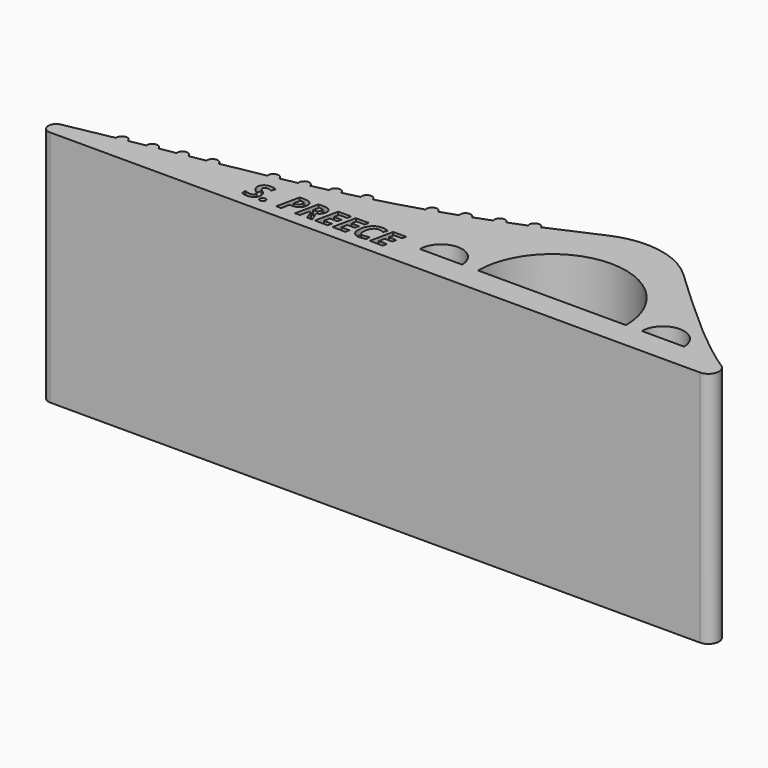
from build123d import *

# Parameters (mm, degrees)
F1_DEPTH     = 45
F2_R         = 1
F3_DEPTH     = 45
F4_TEXT_SIZE = 6.1326831605
F5_DEPTH     = 1


# Not quite as in the source:
# - Text() gives the source's letters only with a copy of the font that has no kerning and outlines rounded to 1/6400 em; it was checked with that copy


with BuildPart() as f1:
    # F0 (on Top) → F1 (new body)
    with BuildSketch(Plane.XY):
        with BuildLine():
            ThreePointArc((-38.2745055444, 2.9746683377), (-39.493653659, 1.3621640586), (-38, 0))
            Line((-38, 0), (85, 0))
            ThreePointArc((85, 0), (86.8753803217, 1.3050549309), (86.3032863072, 3.517051351))
            add(Edge.make_bspline(
                [(63.6094519155, 22.8587176037), (66.2511582833, 20.3082860848), (73.4024087404, 13.801155441), (80.5793521842, 7.3397050188), (86.3032863072, 3.517051351)],
                knots=[0.2378372869, 0.2378372869, 0.2378372869, 0.2378372869, 0.5099450592, 1, 1, 1, 1], degree=3))
            ThreePointArc((63.6094519155, 22.8587176037), (55.7058378489, 26.8549949617), (46.9254964743, 25.6961363077))
            add(Edge.make_bspline(
                [(-38.2745055444, 2.9746683377), (-20.000344137, 6.6962685785), (11.2093039826, 10.6710156773), (37.2235139545, 21.2359519697), (46.9254964743, 25.6961363077)],
                knots=[0, 0, 0, 0, 0.5271651991, 0.8814194919, 0.8814194919, 0.8814194919, 0.8814194919], degree=3))
        make_face()
        with BuildLine():
            Line((36, 5), (28, 5))
            ThreePointArc((28, 5), (32, 9), (36, 5))
        make_face(mode=Mode.SUBTRACT)
        with BuildLine():
            Line((78, 5), (70, 5))
            ThreePointArc((70, 5), (74, 9), (78, 5))
        make_face(mode=Mode.SUBTRACT)
        with BuildLine():
            Line((67, 5), (39, 5))
            ThreePointArc((39, 5), (53, 19), (67, 5))
        make_face(mode=Mode.SUBTRACT)
    extrude(amount=F1_DEPTH)

    # F2 (on face) → F3 (join, through all)
    with BuildSketch(Plane.XY.offset(45)):
        with Locations((-28.2745055444, 4.8948250143)):
            Circle(F2_R)
        with Locations((-23.2745055444, 5.7959024686)):
            Circle(F2_R)
        with Locations((-18.2745055444, 6.6823522477)):
            Circle(F2_R)
        with Locations((-13.2745055444, 7.5727688811)):
            Circle(F2_R)
        with Locations((-3.2745055444, 9.4429018516)):
            Circle(F2_R)
        with Locations((1.7254944556, 10.4641802944)):
            Circle(F2_R)
        with Locations((6.7254944556, 11.5736433304)):
            Circle(F2_R)
        with Locations((11.7254944556, 12.7976294115)):
            Circle(F2_R)
        with Locations((21.7254944556, 15.7002005125)):
            Circle(F2_R)
        with Locations((26.7254944556, 17.3959685149)):
            Circle(F2_R)
        with Locations((31.7254944556, 19.2452773506)):
            Circle(F2_R)
        with Locations((36.7254944556, 21.2381876202)):
            Circle(F2_R)
    extrude(amount=-F3_DEPTH)

    # F4 (on face) → F5 (cut)
    with BuildSketch(Plane.XY.offset(45)):
        with Locations((-3.8470909931, 2.4212112185)):
            Text('S. PREECE', F4_TEXT_SIZE, font='Open Sans', font_style=FontStyle.BOLDITALIC, text_align=(TextAlign.LEFT, TextAlign.BOTTOM))
    extrude(amount=-F5_DEPTH, mode=Mode.SUBTRACT)


solid = f1.part
